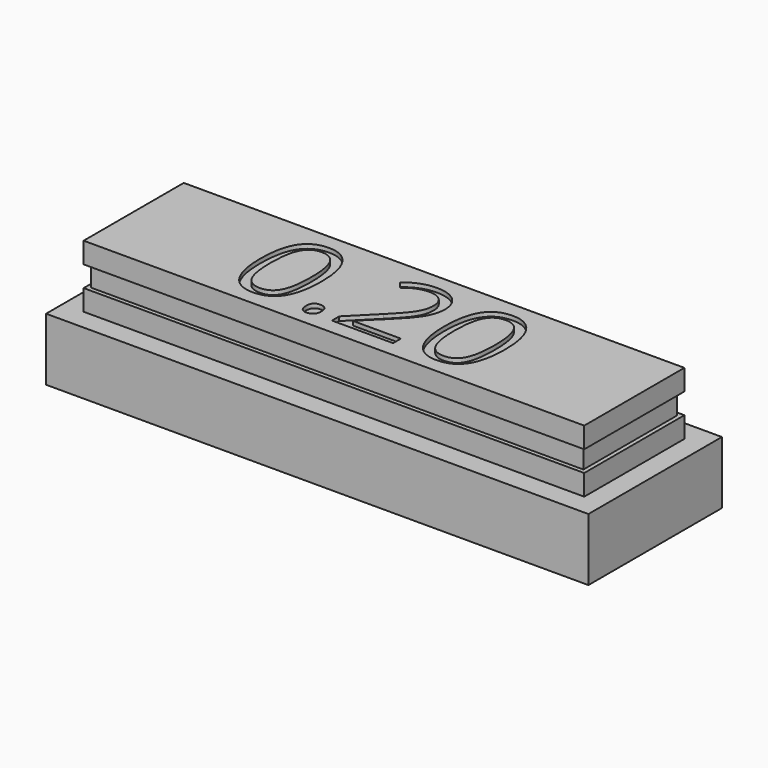
from build123d import *

# Parameters (mm, degrees)
F0_W         = 26
F0_H         = 8
F0_W_2       = 20
F0_H_2       = 2
F1_DEPTH     = 3
F2_W         = 24
F2_H         = 6
F3_DEPTH     = 3
F5_W         = 24
F5_H         = 6
F5_W_2       = 23.6
F5_H_2       = 5.6
F6_DEPTH     = 0.5
F7_W         = 19.6
F7_H         = 1.6
F8_DEPTH     = 3
F9_TEXT_SIZE = 6.25
F10_DEPTH    = 0.2


# Not quite as in the source:
# - Text() gives the source's letters only with a copy of the font that has no kerning and outlines rounded to 1/6400 em; it was checked with that copy


with BuildPart() as f1:
    # F0 (on Top) → F1 (new body)
    with BuildSketch(Plane.XY):
        Rectangle(F0_W, F0_H)
        Rectangle(F0_W_2, F0_H_2, mode=Mode.SUBTRACT)
    extrude(amount=F1_DEPTH)


with BuildPart() as f3:
    # F2 (on face) → F3 (new body)
    with BuildSketch(Plane.XY.offset(3)):
        Rectangle(F2_W, F2_H)
    extrude(amount=F3_DEPTH)

    # F5 (on mid) → F6 (cut, symmetric)
    with BuildSketch(Plane.XY.offset(4.5)):
        Rectangle(F5_W, F5_H)
        Rectangle(F5_W_2, F5_H_2, mode=Mode.SUBTRACT)
    extrude(amount=F6_DEPTH, both=True, mode=Mode.SUBTRACT)

    # F7 (on face) → F8 (join, through all)
    with BuildSketch(Plane(origin=(0, 0, 3), x_dir=(1, 0, 0), z_dir=(0, 0, -1))):
        Rectangle(F7_W, F7_H)
    extrude(amount=F8_DEPTH)

    # F9 (on face) → F10 (cut)
    with BuildSketch(Plane.XY.offset(6)):
        with Locations((-6.2387695312, -2.25)):
            Text('0.20', F9_TEXT_SIZE, font='Open Sans', text_align=(TextAlign.LEFT, TextAlign.BOTTOM))
    extrude(amount=-F10_DEPTH, mode=Mode.SUBTRACT)


solid = Compound([f1.part, f3.part])
